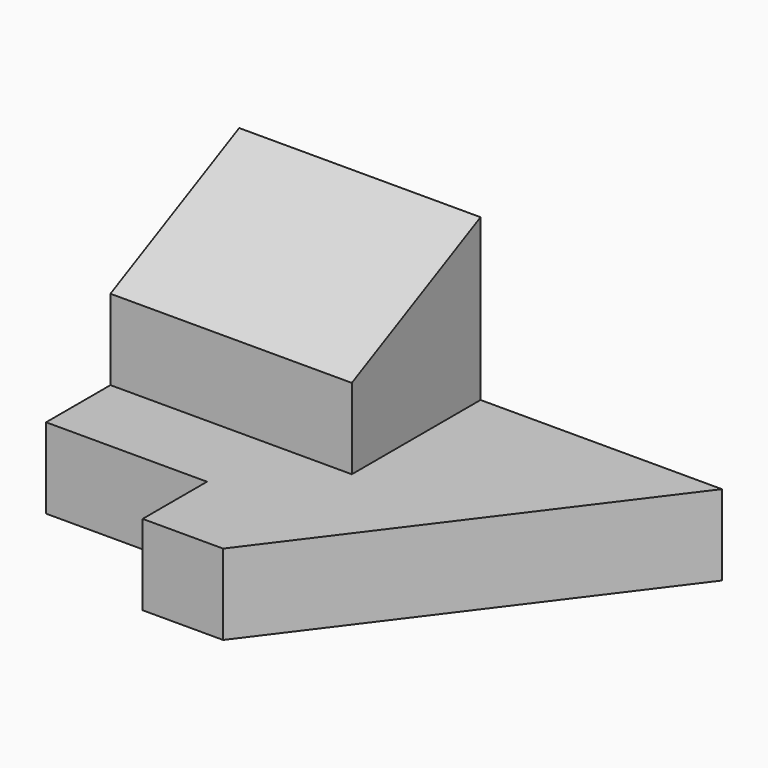
from build123d import *

# Parameters (mm, degrees)
F1_DEPTH = 10
F2_W     = 30
F2_H     = 20
F3_DEPTH = 20
F4_SIZE2 = 9.99999
F4_SIZE  = 19.99999


# Not quite as in the source:
# - a fillet or chamfer is up to 0.001 mm smaller than in the source, because OpenCascade refuses the exact size


with BuildPart() as f1:
    # F0 (on Top) → F1 (new body)
    with BuildSketch(Plane.XY):
        Polygon((0, 30), (0, 0), (20, 0), (20, -10), (30, -10), (60, 30), align=None)
    extrude(amount=F1_DEPTH)

    # F2 (on face) → F3 (join)
    with BuildSketch(Plane.XY.offset(10)):
        with Locations((15, 20)):
            Rectangle(F2_W, F2_H)
    extrude(amount=F3_DEPTH)

    # F4 (size 20 and 10 in the source; OpenCascade refuses exactly that, so slightly less here)
    f4_edges = [f1.edges().sort_by_distance(p)[0] for p in [
        (15, 10, 30),
    ]]
    f4_side = f1.faces().sort_by_distance((15, 20, 30))[0]
    chamfer(f4_edges, length=F4_SIZE, length2=F4_SIZE2, reference=f4_side)


solid = f1.part
